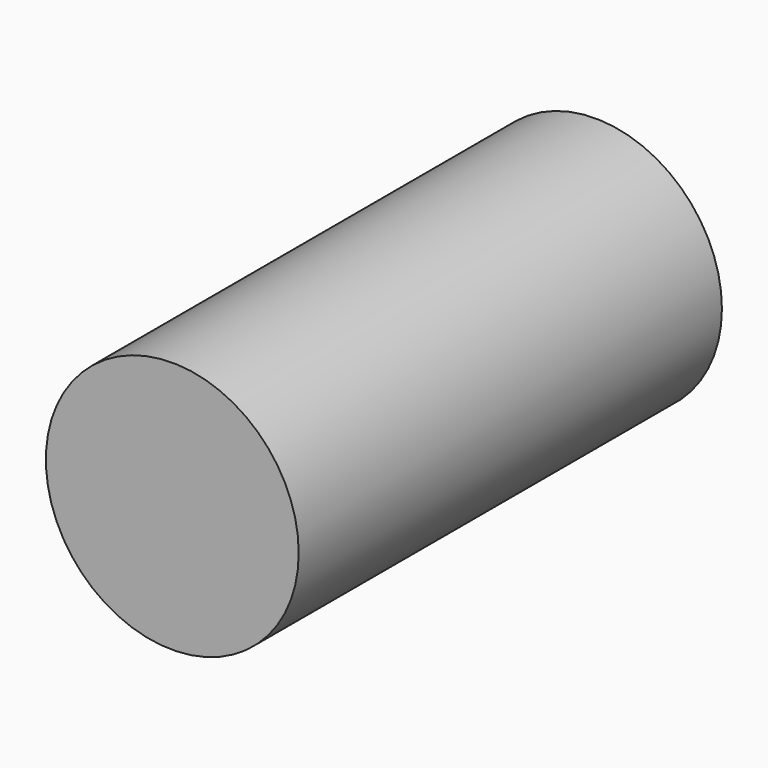
from build123d import *

# Parameters (mm, degrees)
F2_R     = 5.975
F3_DEPTH = 25


# Not quite as in the source:
# - the program builds the solid bodies; features that only make, move or delete a surface that nothing else refers to are left out


with BuildPart() as f3:
    # F2 (on Front) → F3 (new body)
    with BuildSketch(Plane.XZ):
        Circle(F2_R)
    extrude(amount=F3_DEPTH)


solid = f3.part
